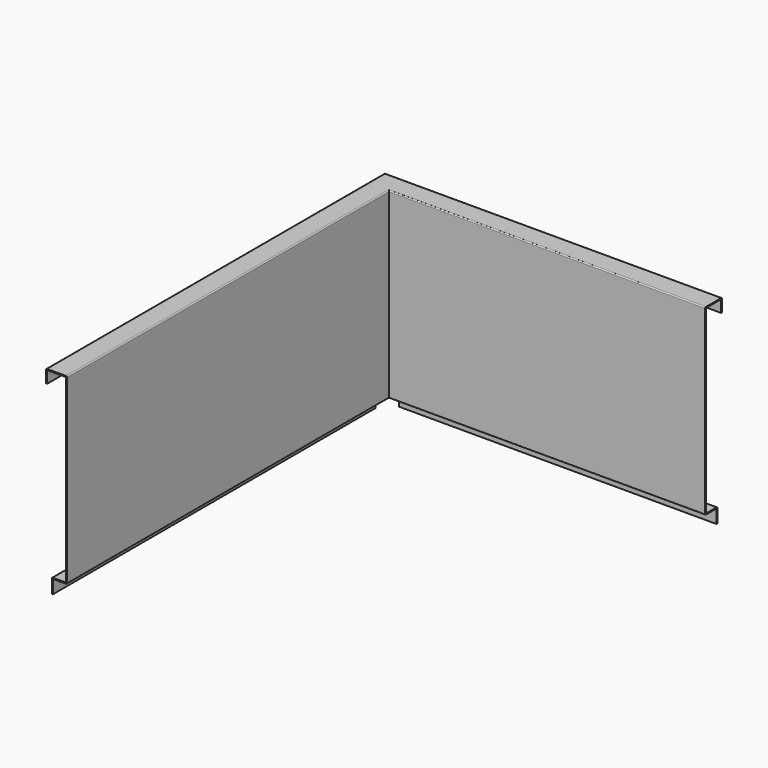
from build123d import *

# Parameters (mm, degrees)
F3_W         = 27
F3_H         = 27
F4_DEPTH     = 30
F5_T1_DEPTH  = 607
F5_T3_DEPTH  = 772
F5_T5_DEPTH  = 808
F5_T7_DEPTH  = 643
F5_T13_DEPTH = 777
F5_T17_DEPTH = 612
F5_T20_DEPTH = 617
F5_T22_DEPTH = 782
F5_T24_DEPTH = 820
F5_T26_DEPTH = 775
F5_T28_DEPTH = 610
F5_T30_DEPTH = 655
F5_T36_DEPTH = 780
F5_T40_DEPTH = 615
F5_T47_DEPTH = 780
F5_T51_DEPTH = 615


# Not quite as in the source:
# - a fillet or chamfer that OpenCascade refuses, or shapes differently, is made with other operations: its cross-section is extruded or revolved along the edge and cut away or added


with BuildPart() as f2:
    # F2: sweep along a path in F1
    with BuildLine(Plane.XY) as f2_path:
        Line((0, 0), (0, 770))
        Line((0, 770), (605, 770))
    # F0 (on Front) → F2 (sweep)
    with BuildSketch(Plane.XZ):
        Polygon((0, -350), (0, 0), (-40, 0), (-40, -25), (-38, -25), (-38, -2), (-2, -2), (-2, -348), (-29, -348), (-29, -376), (-27, -376), (-27, -350), align=None)
    sweep(path=f2_path.line, transition=Transition.RIGHT)

    # F3 (on face) → F4 (cut)
    with BuildSketch(Plane.XY.offset(-348)):
        with Locations((-15.5, 785.5)):
            Rectangle(F3_W, F3_H)
    extrude(amount=-F4_DEPTH, mode=Mode.SUBTRACT)

    # F5: fillet of radius 2 on 15 edges, made by hand

    # F5_s2 → F5_t1 (join)
    with BuildSketch(Plane.YZ.offset(-2)):
        with BuildLine():
            ThreePointArc((774, -348), (772.5857864376, -347.4142135624), (772, -346))
            Line((772, -346), (772, -348))
            Line((772, -348), (774, -348))
        make_face()
        with BuildLine():
            ThreePointArc((774, -2), (772.5857864376, -2.5857864376), (772, -4))
            Line((772, -4), (772, -2))
            Line((772, -2), (774, -2))
        make_face()
        with BuildLine():
            ThreePointArc((795, -350), (796.4142135624, -350.5857864376), (797, -352))
            Line((797, -352), (797, -350))
            Line((797, -350), (795, -350))
        make_face()
    extrude(amount=F5_T1_DEPTH)

    # F5_s4 → F5_t3 (join)
    with BuildSketch(Plane.XZ.offset(-772)):
        with BuildLine():
            ThreePointArc((-4, -2), (-2.5857864376, -2.5857864376), (-2, -4))
            Line((-2, -4), (-2, -2))
            Line((-2, -2), (-4, -2))
        make_face()
        with BuildLine():
            ThreePointArc((-25, -350), (-26.4142135624, -350.5857864376), (-27, -352))
            Line((-27, -352), (-27, -350))
            Line((-27, -350), (-25, -350))
        make_face()
    extrude(amount=F5_T3_DEPTH)

    # F5_s6 → F5_t5 (join)
    with BuildSketch(Plane.XZ.offset(-808)):
        with BuildLine():
            ThreePointArc((-38, -4), (-37.4142135624, -2.5857864376), (-36, -2))
            Line((-36, -2), (-38, -2))
            Line((-38, -2), (-38, -4))
        make_face()
    extrude(amount=F5_T5_DEPTH)

    # F5_s8 → F5_t7 (join)
    with BuildSketch(Plane.YZ.offset(-38)):
        with BuildLine():
            ThreePointArc((806, -2), (807.4142135624, -2.5857864376), (808, -4))
            Line((808, -4), (808, -2))
            Line((808, -2), (806, -2))
        make_face()
    extrude(amount=F5_T7_DEPTH)


with BuildPart() as f5_tool11:
    # F5_s12 → F5_t13 (new body)
    with BuildSketch(Plane.XZ):
        with BuildLine():
            ThreePointArc((-4, -2), (-2.5857864376, -2.5857864376), (-2, -4))
            Line((-2, -4), (-2, -2))
            Line((-2, -2), (-4, -2))
        make_face()
    extrude(amount=-F5_T13_DEPTH)

    split(bisect_by=Plane.XZ.offset(-772), keep=Keep.BOTTOM)


with BuildPart() as f5_tool15:
    # F5_s16 → F5_t17 (new body)
    with BuildSketch(Plane.YZ.offset(-7)):
        with BuildLine():
            ThreePointArc((774, -2), (772.5857864376, -2.5857864376), (772, -4))
            Line((772, -4), (772, -2))
            Line((772, -2), (774, -2))
        make_face()
    extrude(amount=F5_T17_DEPTH)

    split(bisect_by=Plane.YZ.offset(-2), keep=Keep.BOTTOM)


with BuildPart() as f5_tool11_1:
    add(f5_tool11.part)

    # F5_t19: intersect F5_tool15
    add(f5_tool15.part, mode=Mode.INTERSECT)


with BuildPart() as f2_1:
    add(f2.part)

    # F5_t9: union F5_tool11
    add(f5_tool11_1.part)

    # F5_s21 → F5_t20 (cut)
    with BuildSketch(Plane.YZ.offset(-7)):
        with BuildLine():
            ThreePointArc((799, -350), (798.4142135624, -348.5857864376), (797, -348))
            Line((797, -348), (799, -348))
            Line((799, -348), (799, -350))
        make_face()
    extrude(amount=F5_T20_DEPTH, mode=Mode.SUBTRACT)

    # F5_s23 → F5_t22 (cut)
    with BuildSketch(Plane.XZ.offset(-777)):
        with BuildLine():
            ThreePointArc((-29, -350), (-28.4142135624, -348.5857864376), (-27, -348))
            Line((-27, -348), (-29, -348))
            Line((-29, -348), (-29, -350))
        make_face()
    extrude(amount=F5_T22_DEPTH, mode=Mode.SUBTRACT)

    # F5_s25 → F5_t24 (cut)
    with BuildSketch(Plane.XZ.offset(-815)):
        with BuildLine():
            ThreePointArc((-40, -2), (-39.4142135624, -0.5857864376), (-38, 0))
            Line((-38, 0), (-40, 0))
            Line((-40, 0), (-40, -2))
        make_face()
    extrude(amount=F5_T24_DEPTH, mode=Mode.SUBTRACT)

    # F5_s27 → F5_t26 (cut)
    with BuildSketch(Plane.XZ.offset(-770)):
        with BuildLine():
            ThreePointArc((0, -2), (-0.5857864376, -0.5857864376), (-2, 0))
            Line((-2, 0), (0, 0))
            Line((0, 0), (0, -2))
        make_face()
        with BuildLine():
            ThreePointArc((0, -348), (-0.5857864376, -349.4142135624), (-2, -350))
            Line((-2, -350), (0, -350))
            Line((0, -350), (0, -348))
        make_face()
    extrude(amount=F5_T26_DEPTH, mode=Mode.SUBTRACT)

    # F5_s29 → F5_t28 (cut)
    with BuildSketch(Plane.YZ):
        with BuildLine():
            ThreePointArc((770, -2), (770.5857864376, -0.5857864376), (772, 0))
            Line((772, 0), (770, 0))
            Line((770, 0), (770, -2))
        make_face()
        with BuildLine():
            ThreePointArc((770, -348), (770.5857864376, -349.4142135624), (772, -350))
            Line((772, -350), (770, -350))
            Line((770, -350), (770, -348))
        make_face()
    extrude(amount=F5_T28_DEPTH, mode=Mode.SUBTRACT)

    # F5_s31 → F5_t30 (cut)
    with BuildSketch(Plane.YZ.offset(-45)):
        with BuildLine():
            ThreePointArc((810, -2), (809.4142135624, -0.5857864376), (808, 0))
            Line((808, 0), (810, 0))
            Line((810, 0), (810, -2))
        make_face()
    extrude(amount=F5_T30_DEPTH, mode=Mode.SUBTRACT)


with BuildPart() as f5_tool34:
    # F5_s35 → F5_t36 (new body)
    with BuildSketch(Plane.XZ.offset(5)):
        with BuildLine():
            ThreePointArc((0, -2), (-0.5857864376, -0.5857864376), (-2, 0))
            Line((-2, 0), (0, 0))
            Line((0, 0), (0, -2))
        make_face()
    extrude(amount=-F5_T36_DEPTH)

    split(bisect_by=Plane.XZ.offset(-770), keep=Keep.BOTTOM)


with BuildPart() as f5_tool38:
    # F5_s39 → F5_t40 (new body)
    with BuildSketch(Plane.YZ.offset(-5)):
        with BuildLine():
            ThreePointArc((770, -2), (770.5857864376, -0.5857864376), (772, 0))
            Line((772, 0), (770, 0))
            Line((770, 0), (770, -2))
        make_face()
    extrude(amount=F5_T40_DEPTH)

    split(bisect_by=Plane.YZ, keep=Keep.BOTTOM)


with BuildPart() as f5_tool34_1:
    add(f5_tool34.part)

    # F5_t42: intersect F5_tool38
    add(f5_tool38.part, mode=Mode.INTERSECT)


with BuildPart() as f2_2:
    add(f2_1.part)

    # F5_t32: cut F5_tool34
    add(f5_tool34_1.part, mode=Mode.SUBTRACT)


with BuildPart() as f5_tool45:
    # F5_s46 → F5_t47 (new body)
    with BuildSketch(Plane.XZ.offset(5)):
        with BuildLine():
            ThreePointArc((0, -348), (-0.5857864376, -349.4142135624), (-2, -350))
            Line((-2, -350), (0, -350))
            Line((0, -350), (0, -348))
        make_face()
    extrude(amount=-F5_T47_DEPTH)

    split(bisect_by=Plane.XZ.offset(-770), keep=Keep.BOTTOM)


with BuildPart() as f5_tool49:
    # F5_s50 → F5_t51 (new body)
    with BuildSketch(Plane.YZ.offset(-5)):
        with BuildLine():
            ThreePointArc((770, -348), (770.5857864376, -349.4142135624), (772, -350))
            Line((772, -350), (770, -350))
            Line((770, -350), (770, -348))
        make_face()
    extrude(amount=F5_T51_DEPTH)

    split(bisect_by=Plane.YZ, keep=Keep.BOTTOM)


with BuildPart() as f5_tool45_1:
    add(f5_tool45.part)

    # F5_t53: intersect F5_tool49
    add(f5_tool49.part, mode=Mode.INTERSECT)


with BuildPart() as f2_3:
    add(f2_2.part)

    # F5_t43: cut F5_tool45
    add(f5_tool45_1.part, mode=Mode.SUBTRACT)


solid = f2_3.part
